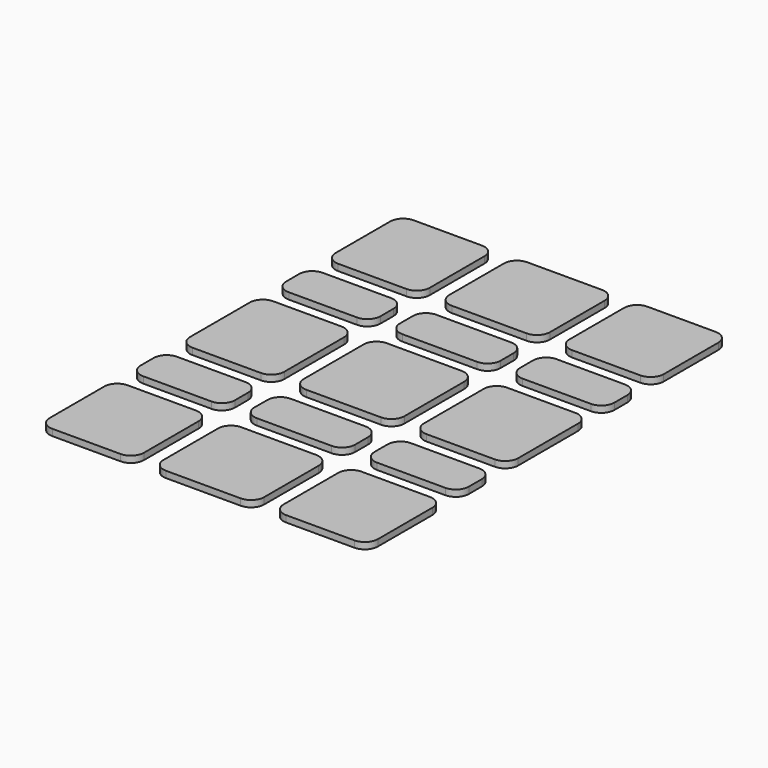
from build123d import *

# Parameters (mm, degrees)
F1_DEPTH = 1


with BuildPart() as f1:
    # F0 (on Top) → F1 (new body)
    with BuildSketch(Plane.XY):
        with BuildLine():
            ThreePointArc((7.75, 5.75), (7.1642135624, 7.1642135624), (5.75, 7.75))
            Line((5.75, 7.75), (-5.75, 7.75))
            ThreePointArc((-5.75, 7.75), (-7.1642135624, 7.1642135624), (-7.75, 5.75))
            Line((-7.75, 5.75), (-7.75, -5.75))
            ThreePointArc((-7.75, -5.75), (-7.1642135624, -7.1642135624), (-5.75, -7.75))
            Line((-5.75, -7.75), (5.75, -7.75))
            ThreePointArc((5.75, -7.75), (7.1642135624, -7.1642135624), (7.75, -5.75))
            Line((7.75, -5.75), (7.75, 5.75))
        make_face()
    extrude(amount=F1_DEPTH)


with BuildPart() as f1b:
    # F0 (on Top) → F1, piece 2 (new body)
    with BuildSketch(Plane.XY):
        with BuildLine():
            Line((5.75, -10.75), (-5.75, -10.75))
            ThreePointArc((-5.75, -10.75), (-7.1642135624, -11.3357864376), (-7.75, -12.75))
            Line((-7.75, -12.75), (-7.75, -15.25))
            ThreePointArc((-7.75, -15.25), (-7.1642135624, -16.6642135624), (-5.75, -17.25))
            Line((-5.75, -17.25), (5.75, -17.25))
            ThreePointArc((5.75, -17.25), (7.1642135624, -16.6642135624), (7.75, -15.25))
            Line((7.75, -15.25), (7.75, -12.75))
            ThreePointArc((7.75, -12.75), (7.1642135624, -11.3357864376), (5.75, -10.75))
        make_face()
    extrude(amount=F1_DEPTH)


with BuildPart() as f1c:
    # F0 (on Top) → F1, piece 3 (new body)
    with BuildSketch(Plane.XY):
        with BuildLine():
            ThreePointArc((-10.75, 5.75), (-11.3357864376, 7.1642135624), (-12.75, 7.75))
            Line((-12.75, 7.75), (-23.25, 7.75))
            ThreePointArc((-23.25, 7.75), (-24.6642135624, 7.1642135624), (-25.25, 5.75))
            Line((-25.25, 5.75), (-25.25, -5.75))
            ThreePointArc((-25.25, -5.75), (-24.6642135624, -7.1642135624), (-23.25, -7.75))
            Line((-23.25, -7.75), (-12.75, -7.75))
            ThreePointArc((-12.75, -7.75), (-11.3357864376, -7.1642135624), (-10.75, -5.75))
            Line((-10.75, -5.75), (-10.75, 5.75))
        make_face()
    extrude(amount=F1_DEPTH)


with BuildPart() as f1d:
    # F0 (on Top) → F1, piece 4 (new body)
    with BuildSketch(Plane.XY):
        with BuildLine():
            Line((-12.75, -10.75), (-23.25, -10.75))
            ThreePointArc((-23.25, -10.75), (-24.6642135624, -11.3357864376), (-25.25, -12.75))
            Line((-25.25, -12.75), (-25.25, -15.25))
            ThreePointArc((-25.25, -15.25), (-24.6642135624, -16.6642135624), (-23.25, -17.25))
            Line((-23.25, -17.25), (-12.75, -17.25))
            ThreePointArc((-12.75, -17.25), (-11.3357864376, -16.6642135624), (-10.75, -15.25))
            Line((-10.75, -15.25), (-10.75, -12.75))
            ThreePointArc((-10.75, -12.75), (-11.3357864376, -11.3357864376), (-12.75, -10.75))
        make_face()
    extrude(amount=F1_DEPTH)


with BuildPart() as f1e:
    # F0 (on Top) → F1, piece 5 (new body)
    with BuildSketch(Plane.XY):
        with BuildLine():
            Line((-12.75, -20.25), (-23.25, -20.25))
            ThreePointArc((-23.25, -20.25), (-24.6642135624, -20.8357864376), (-25.25, -22.25))
            Line((-25.25, -22.25), (-25.25, -32.75))
            ThreePointArc((-25.25, -32.75), (-24.6642135624, -34.1642135624), (-23.25, -34.75))
            Line((-23.25, -34.75), (-12.75, -34.75))
            ThreePointArc((-12.75, -34.75), (-11.3357864376, -34.1642135624), (-10.75, -32.75))
            Line((-10.75, -32.75), (-10.75, -22.25))
            ThreePointArc((-10.75, -22.25), (-11.3357864376, -20.8357864376), (-12.75, -20.25))
        make_face()
    extrude(amount=F1_DEPTH)


with BuildPart() as f1f:
    # F0 (on Top) → F1, piece 6 (new body)
    with BuildSketch(Plane.XY):
        with BuildLine():
            Line((5.75, -20.25), (-5.75, -20.25))
            ThreePointArc((-5.75, -20.25), (-7.1642135624, -20.8357864376), (-7.75, -22.25))
            Line((-7.75, -22.25), (-7.75, -32.75))
            ThreePointArc((-7.75, -32.75), (-7.1642135624, -34.1642135624), (-5.75, -34.75))
            Line((-5.75, -34.75), (5.75, -34.75))
            ThreePointArc((5.75, -34.75), (7.1642135624, -34.1642135624), (7.75, -32.75))
            Line((7.75, -32.75), (7.75, -22.25))
            ThreePointArc((7.75, -22.25), (7.1642135624, -20.8357864376), (5.75, -20.25))
        make_face()
    extrude(amount=F1_DEPTH)


with BuildPart() as f2_1:
    # F2: instance of F1c
    add(f1c.part.mirror(Plane.YZ))


with BuildPart() as f2_2:
    # F2: instance of F1d
    add(f1d.part.mirror(Plane.YZ))


with BuildPart() as f2_3:
    # F2: instance of F1e
    add(f1e.part.mirror(Plane.YZ))


with BuildPart() as f3_1:
    # F3: instance of F1d
    add(f1d.part.mirror(Plane.XZ))


with BuildPart() as f3_2:
    # F3: instance of F1e
    add(f1e.part.mirror(Plane.XZ))


with BuildPart() as f3_3:
    # F3: instance of F1f
    add(f1f.part.mirror(Plane.XZ))


with BuildPart() as f3_4:
    # F3: instance of F1b
    add(f1b.part.mirror(Plane.XZ))


with BuildPart() as f3_5:
    # F3: instance of F2_2
    add(f2_2.part.mirror(Plane.XZ))


with BuildPart() as f3_6:
    # F3: instance of F2_3
    add(f2_3.part.mirror(Plane.XZ))


solid = Compound([f1.part, f1b.part, f1c.part, f1d.part, f1e.part, f1f.part, f2_1.part, f2_2.part, f2_3.part, f3_1.part, f3_2.part, f3_3.part, f3_4.part, f3_5.part, f3_6.part])
